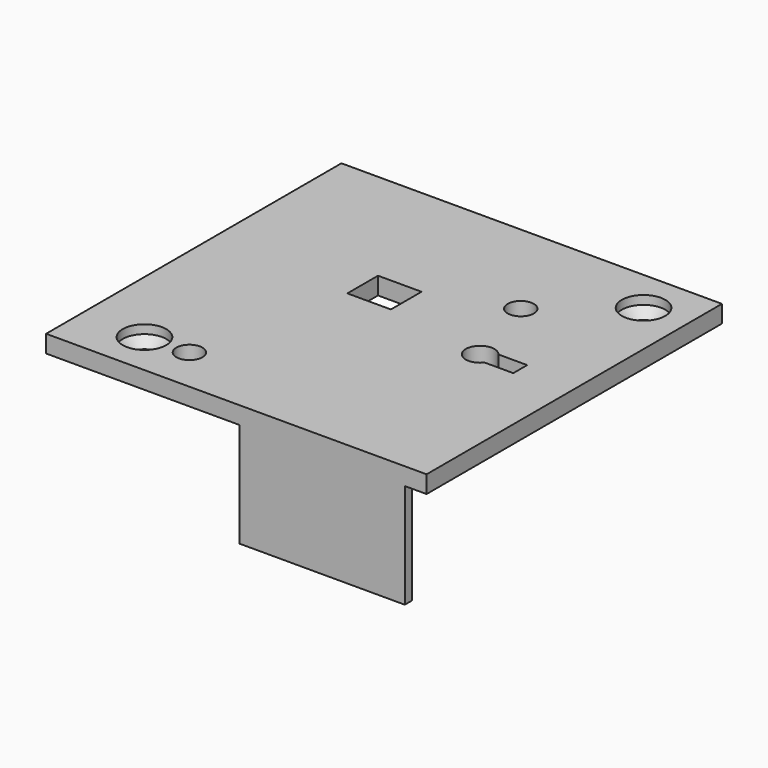
from build123d import *

# Parameters (mm, degrees)
F1_W     = 43.7
F1_H     = 42.4
F1_R     = 1.5
F1_W_2   = 5
F1_H_2   = 4.4
F2_DEPTH = 1
F3_SIZE  = 0.99999
F4_DEPTH = 1
F5_W     = 19
F5_H     = 1
F6_DEPTH = 12


# Not quite as in the source:
# - a fillet or chamfer is up to 0.001 mm smaller than in the source, because OpenCascade refuses the exact size


with BuildPart() as f2:
    # F1 (on face) → F2 (new body)
    with BuildSketch(Plane.XY):
        with Locations((-38.7602308843, 29.1194021702)):
            Rectangle(F1_W, F1_H)
        with Locations((-53.3102308843, 12.9194021702)):
            Circle(F1_R, mode=Mode.SUBTRACT)
        with Locations((-48.3102308843, 13.1194021702)):
            Circle(F1_R, mode=Mode.SUBTRACT)
        with Locations((-41.9102308843, 33.1194021702)):
            Rectangle(F1_W_2, F1_H_2, mode=Mode.SUBTRACT)
        with Locations((-30.4102308843, 38.3194021702)):
            Circle(F1_R, mode=Mode.SUBTRACT)
        with BuildLine():
            ThreePointArc((-26.4145926142, 28.1194021702), (-29.3713070947, 29.1194021702), (-26.4145926142, 30.1194021702))
            Line((-26.4145926142, 30.1194021702), (-23.1138560921, 30.1194021702))
            Line((-23.1138560921, 30.1194021702), (-23.1138560921, 28.1194021702))
            Line((-23.1138560921, 28.1194021702), (-26.4145926142, 28.1194021702))
        make_face(mode=Mode.SUBTRACT)
        with Locations((-21.9102308843, 45.3194021702)):
            Circle(F1_R, mode=Mode.SUBTRACT)
    extrude(amount=F2_DEPTH)

    # F3 (size 1 in the source; OpenCascade refuses exactly that, so slightly less here)
    f3_edges = [f2.edges().sort_by_distance(p)[0] for p in [
        (-23.410231, 45.319402, 1),
        (-54.810231, 12.919402, 1),
    ]]
    chamfer(f3_edges, length=F3_SIZE)

    # F4 (add): a face of the model
    f4_faces = [f2.faces().sort_by_distance(p)[0] for p in [
        (-38.8442562914, 29.0967487251, 1),
    ]]
    extrude(f4_faces, amount=F4_DEPTH)

    # F5 (on face) → F6 (join)
    with BuildSketch(Plane.XY):
        with Locations((-28.9102308843, 8.4194021702)):
            Rectangle(F5_W, F5_H)
    extrude(amount=-F6_DEPTH)


solid = f2.part
